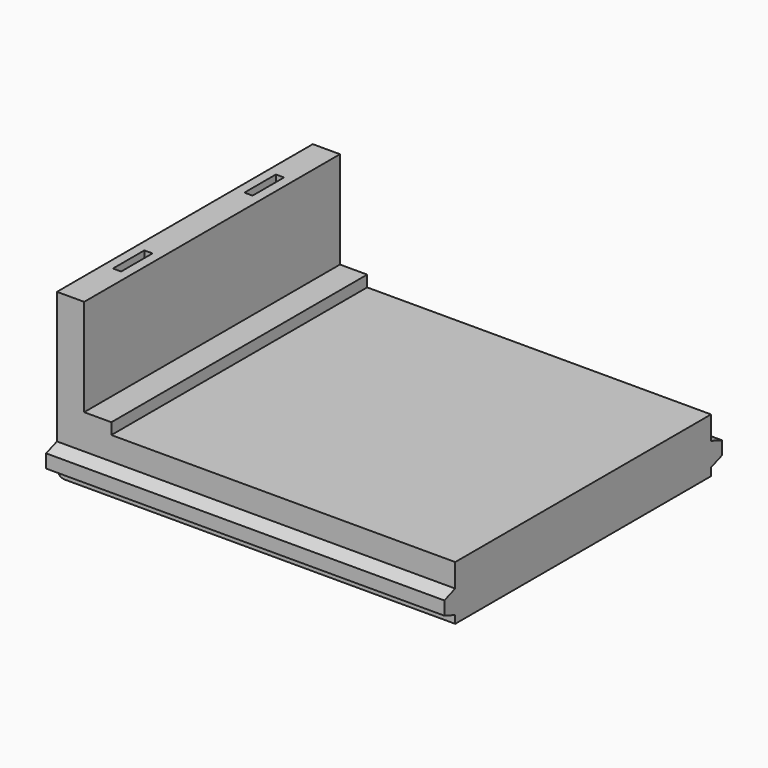
from build123d import *

# Parameters (mm, degrees)
F0_W         = 102.5
F0_H         = 82.3
F1_DEPTH     = 14
F2_W         = 7
F2_H         = 82.3
F3_DEPTH     = 27.9
F4_W         = 7
F4_H         = 82.3
F5_DEPTH     = 2.9
F7_DEPTH     = 102.5
F8_R         = 2
F11_DEPTH    = 2
F12_T1_DEPTH = 67.5
F12_T4_ANGLE = 180
F12_T6_ANGLE = 180
F13_W        = 2.1
F13_H        = 10.1
F14_DEPTH    = 19.95
F15_R        = 5.04999
F16_R        = 5.04999


# Not quite as in the source:
# - a fillet or chamfer that OpenCascade refuses, or shapes differently, is made with other operations: its cross-section is extruded or revolved along the edge and cut away or added
# - a fillet or chamfer is up to 0.001 mm smaller than in the source, because OpenCascade refuses the exact size


with BuildPart() as f1:
    # F0 (on Top) → F1 (new body)
    with BuildSketch(Plane.XY):
        Rectangle(F0_W, F0_H)
    extrude(amount=F1_DEPTH)

    # F2 (on face) → F3 (join)
    with BuildSketch(Plane.XY.offset(14)):
        with Locations((-47.75, 0)):
            Rectangle(F2_W, F2_H)
    extrude(amount=F3_DEPTH)

    # F4 (on face) → F5 (join)
    with BuildSketch(Plane.XY.offset(14)):
        with Locations((-40.75, 0)):
            Rectangle(F4_W, F4_H)
    extrude(amount=F5_DEPTH)

    # F6 (on face) → F7 (join)
    with BuildSketch(Plane.YZ.offset(51.25)):
        Polygon((41.15, 8), (41.15, 2), (44.65, 3.2738958199), (44.65, 6.7261041801), align=None)
        Polygon((-44.65, 3.2738958199), (-41.15, 2), (-41.15, 8), (-44.65, 6.7261041801), align=None)
    extrude(amount=-F7_DEPTH)

    # F8
    f8_edges = [f1.edges().sort_by_distance(p)[0] for p in [
        (-51.25, 0, 0),
    ]]
    fillet(f8_edges, radius=F8_R)

    # F10: union 

    # F9 (on face) → F11 (cut)
    with BuildSketch(Plane(origin=(0, 0, 0), x_dir=(1, 0, 0), z_dir=(0, 0, -1))):
        with BuildLine():
            ThreePointArc((-24.25, 33.65), (-26.75, 36.15), (-29.25, 33.65))
            Line((-29.25, 33.65), (-29.25, -33.85))
            ThreePointArc((-29.25, -33.85), (-26.75, -36.35), (-24.25, -33.85))
            Line((-24.25, -33.85), (-24.25, 33.65))
        make_face()
    extrude(amount=-F11_DEPTH, mode=Mode.SUBTRACT)

    # F12: fillet of radius 2.2 on 2 edges, made by hand

    # F12_s2 → F12_t1 (join)
    with BuildSketch(Plane.XZ.offset(-33.85)):
        with BuildLine():
            ThreePointArc((-29.25, 0), (-28.5423494674, 1.4248076809), (-27.05910977, 2))
            Line((-27.05910977, 2), (-29.25, 2))
            Line((-29.25, 2), (-29.25, 0))
        make_face()
        with BuildLine():
            ThreePointArc((-24.25, 0), (-24.9576505326, 1.4248076809), (-26.44089023, 2))
            Line((-26.44089023, 2), (-24.25, 2))
            Line((-24.25, 2), (-24.25, 0))
        make_face()
    extrude(amount=F12_T1_DEPTH)

    # F12_s3 → F12_t4 (revolve)
    with BuildSketch(Plane.XZ.offset(-33.85)):
        with BuildLine():
            ThreePointArc((-29.25, 0), (-28.5423494674, 1.4248076809), (-27.05910977, 2))
            Line((-27.05910977, 2), (-29.25, 2))
            Line((-29.25, 2), (-29.25, 0))
        make_face()
    revolve(axis=Axis((-26.75, 33.85, 2), (0, 0, -1)), revolution_arc=F12_T4_ANGLE)

    # F12_s5 → F12_t6 (revolve)
    with BuildSketch(Plane.XZ.offset(33.65)):
        with BuildLine():
            ThreePointArc((-24.25, 0), (-24.9576505326, 1.4248076809), (-26.44089023, 2))
            Line((-26.44089023, 2), (-24.25, 2))
            Line((-24.25, 2), (-24.25, 0))
        make_face()
    revolve(axis=Axis((-26.75, -33.65, 2), (0, 0, -1)), revolution_arc=F12_T6_ANGLE)

    # F13 (on face) → F14 (cut)
    with BuildSketch(Plane.XY.offset(41.9)):
        with Locations((-47.75, 21.15)):
            Rectangle(F13_W, F13_H)
        with Locations((-47.75, -21.15)):
            Rectangle(F13_W, F13_H)
    extrude(amount=-F14_DEPTH, mode=Mode.SUBTRACT)

    # F15 (radius 5.05 in the source; OpenCascade refuses exactly that, so slightly less here)
    f15_edges = [f1.edges().sort_by_distance(p)[0] for p in [
        (-47.75, 16.1, 21.95),
        (-47.75, 26.2, 21.95),
    ]]
    fillet(f15_edges, radius=F15_R)

    # F16 (radius 5.05 in the source; OpenCascade refuses exactly that, so slightly less here)
    f16_edges = [f1.edges().sort_by_distance(p)[0] for p in [
        (-47.75, -16.1, 21.95),
        (-47.75, -26.2, 21.95),
    ]]
    fillet(f16_edges, radius=F16_R)


solid = f1.part
